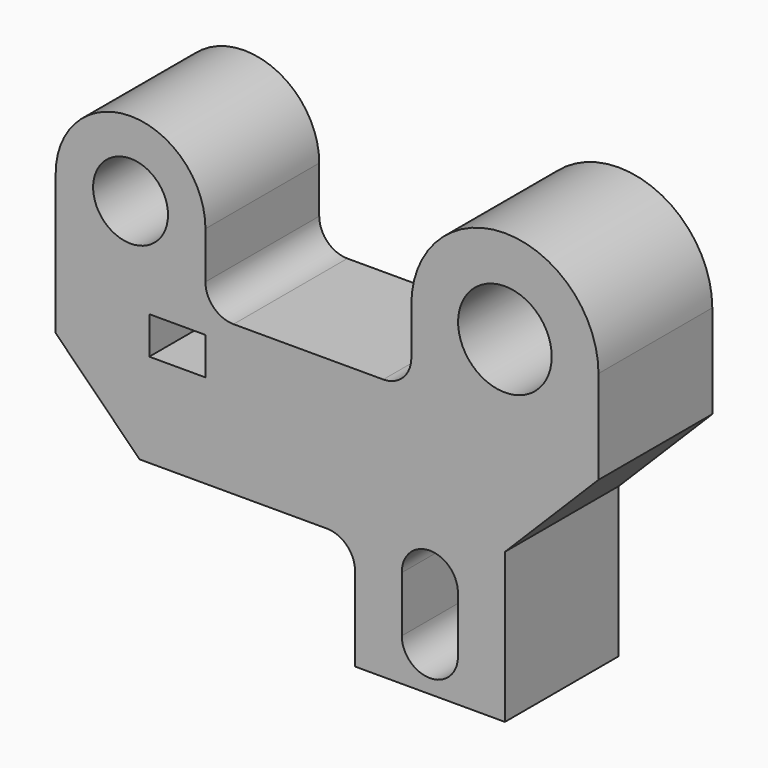
from build123d import *

# Parameters (mm, degrees)
F0_W     = 0.75
F0_H     = 0.5
F0_R     = 0.5
F0_R_2   = 0.625
F1_DEPTH = 1.9


# Not quite as in the source:
# - ends of sketch curves that miss each other by under 0.0002 mm in the source are joined


with BuildPart() as f1:
    # F0 (on Front) → F1 (new body)
    with BuildSketch(Plane.XZ):
        with BuildLine():
            Line((0.0021614751, 1.1225641938), (1.122697085, 0.0020285839))
            Line((1.122697085, 0.0020285839), (3.625, 0.0020285839))
            ThreePointArc((3.625, 0.0020285839), (3.8901650429, -0.1078063731), (4, -0.3729714161))
            Line((4, -0.3729714161), (4, -1.4979714161))
            Line((4, -1.4979714161), (6.0021614751, -1.4979714161))
            Line((6.0021614751, -1.4979714161), (6.0021614751, 0.5020285839))
            Line((6.0021614751, 0.5020285839), (7.2521614751, 1.7551845998))
            Line((7.2521614751, 1.7551845998), (7.2521614751, 3))
            Line((7.2521614751, 3), (7.2521614751, 3.0051845998))
            ThreePointArc((7.2521614751, 3.0051845998), (5.9995691919, 4.249997312), (4.7521614751, 3))
            Line((4.7521614751, 3), (4.7521614751, 2.375))
            ThreePointArc((4.7521614751, 2.375), (4.642326518, 2.1098349571), (4.3771614751, 2))
            Line((4.3771614751, 2), (2.3771614751, 2))
            ThreePointArc((2.3771614751, 2), (2.1119964322, 2.1098349571), (2.0021614751, 2.375))
            Line((2.0021614751, 2.375), (2.0021614751, 3))
            ThreePointArc((2.0021614751, 3), (1.0021614751, 4), (0.0021614751, 3))
            Line((0.0021614751, 3), (0.0021614751, 1.1225641938))
        make_face()
        with BuildLine():
            ThreePointArc((5.3746090938, -0.9511214132), (4.9914239554, -1.3089053091), (4.6250000012, -0.9339737791))
            Line((4.6250000012, -0.9339737791), (4.6250586901, -0.1906377023))
            ThreePointArc((4.6250586901, -0.1906377023), (5.0052444867, 0.1909599387), (5.3746090938, -0.2011214132))
            Line((5.3746090938, -0.2011214132), (5.3746090938, -0.9168853601))
            ThreePointArc((5.3746090938, -0.9168853601), (5.375, -0.9340033866), (5.3746090938, -0.9511214132))
        make_face(mode=Mode.SUBTRACT)
        with Locations((1.6271614751, 1.5020285839)):
            Rectangle(F0_W, F0_H, mode=Mode.SUBTRACT)
        with Locations((1.0021614751, 3)):
            Circle(F0_R, mode=Mode.SUBTRACT)
        with Locations((6.0021614751, 3)):
            Circle(F0_R_2, mode=Mode.SUBTRACT)
    extrude(amount=F1_DEPTH)


solid = f1.part
